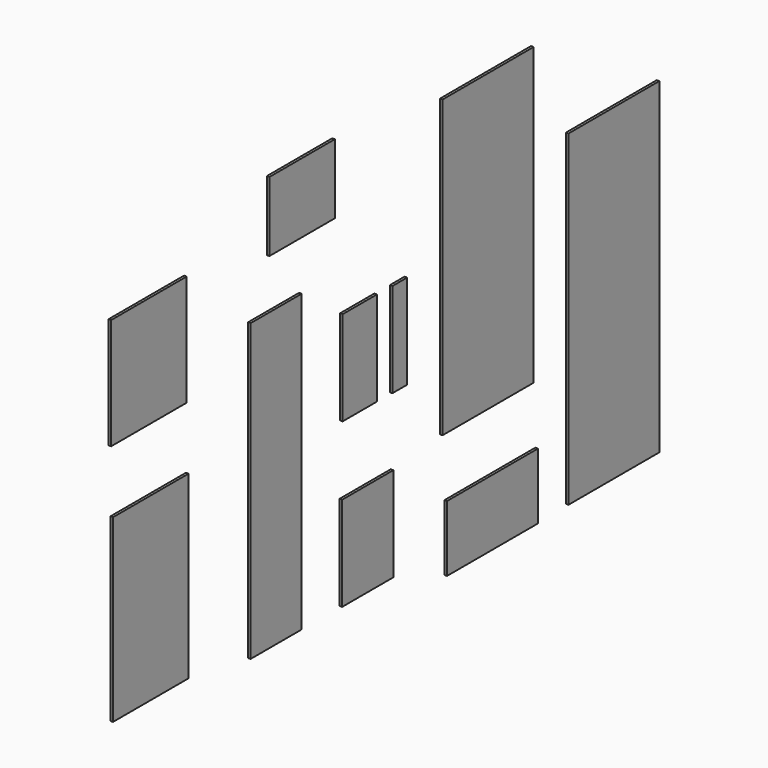
from build123d import *

# Parameters (mm, degrees)
F0_W     = 450
F0_H     = 2080
F1_DEPTH = 18
F0_H_2   = 664
F0_W_2   = 800
F0_H_3   = 2300
F0_W_3   = 664
F0_H_4   = 1268
F0_H_5   = 464
F0_H_6   = 782
F0_W_4   = 302
F0_W_5   = 130
F0_W_6   = 575
F0_H_7   = 490


# Not quite as in the source:
# - a feature names something its author has since deleted; it is built from what else it names


with BuildPart() as f1:
    # F0 (on Right) → F1 (new body)
    with BuildSketch(Plane.YZ):
        with Locations((-1502.587223053, 255.1411771774)):
            Rectangle(F0_W, F0_H)
    extrude(amount=F1_DEPTH)


with BuildPart() as f1b:
    # F0 (on Right) → F1, piece 2 (new body)
    with BuildSketch(Plane.YZ):
        with Locations((-696.9352006912, -457.6543741226)):
            Rectangle(F0_W, F0_H_2)
    extrude(amount=F1_DEPTH)


with BuildPart() as f1c:
    # F0 (on Right) → F1, piece 3 (new body)
    with BuildSketch(Plane.YZ):
        with Locations((361.1036155, 954.3668979353)):
            Rectangle(F0_W_2, F0_H)
    extrude(amount=F1_DEPTH)


with BuildPart() as f1d:
    # F0 (on Right) → F1, piece 4 (new body)
    with BuildSketch(Plane.YZ):
        with Locations((1468.146109581, 183.5974693298)):
            Rectangle(F0_W_2, F0_H_3)
    extrude(amount=F1_DEPTH)


with BuildPart() as f1e:
    # F0 (on Right) → F1, piece 5 (new body)
    with BuildSketch(Plane.YZ):
        with Locations((-2604.9928836823, -48.9639673233)):
            Rectangle(F0_W_3, F0_H_4)
    extrude(amount=F1_DEPTH)


with BuildPart() as f1f:
    # F0 (on Right) → F1, piece 6 (new body)
    with BuildSketch(Plane.YZ):
        with Locations((400, -740.8659391403)):
            Rectangle(F0_W_2, F0_H_5)
    extrude(amount=F1_DEPTH)


with BuildPart() as f1g:
    # F0 (on Right) → F1, piece 7 (new body)
    with BuildSketch(Plane.YZ):
        with Locations((-2621.2816410065, 1421.9926271439)):
            Rectangle(F0_W_3, F0_H_6)
    extrude(amount=F1_DEPTH)


with BuildPart() as f1h:
    # F0 (on Right) → F1, piece 8 (new body)
    with BuildSketch(Plane.YZ):
        with Locations((-766.6916480064, 689.7170372009)):
            Rectangle(F0_W_4, F0_H_2)
    extrude(amount=F1_DEPTH)


with BuildPart() as f1i:
    # F0 (on Right) → F1, piece 9 (new body)
    with BuildSketch(Plane.YZ):
        with Locations((-414.567438364, 686.1258871555)):
            Rectangle(F0_W_5, F0_H_2)
    extrude(amount=F1_DEPTH)


with BuildPart() as f1j:
    # F0 (on Right) → F1, piece 10 (new body)
    with BuildSketch(Plane.YZ):
        with Locations((-1274.1632699966, 1888.6480283737)):
            Rectangle(F0_W_6, F0_H_7)
    extrude(amount=F1_DEPTH)


solid = Compound([f1.part, f1b.part, f1c.part, f1d.part, f1e.part, f1f.part, f1g.part, f1h.part, f1i.part, f1j.part])
